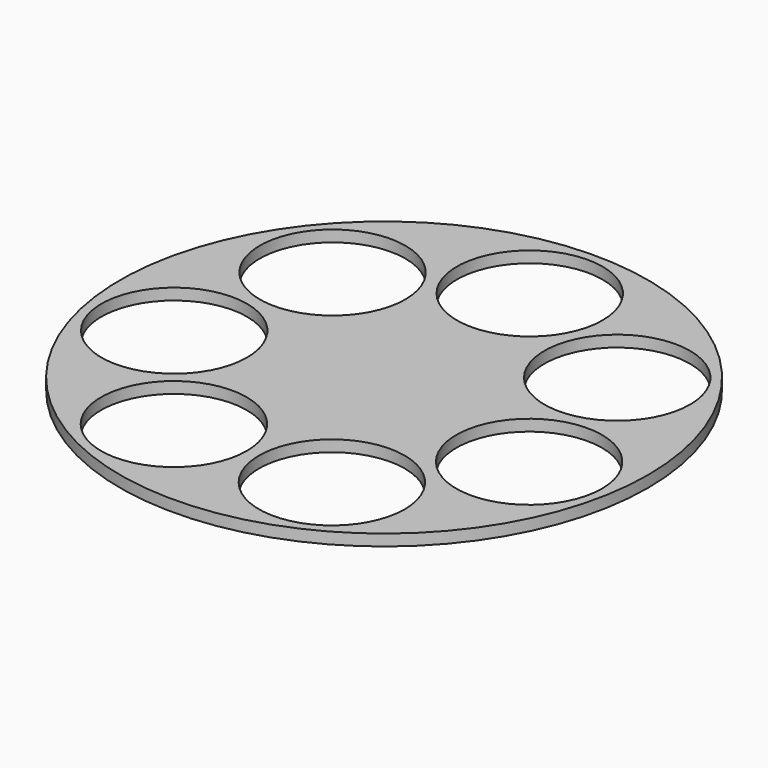
from build123d import *

# Parameters (mm, degrees)
F0_R     = 116
F0_R_2   = 32
F2_DEPTH = 5


# Not quite as in the source:
# - the program builds the solid bodies; features that only make, move or delete a surface that nothing else refers to are left out


with BuildPart() as f2:
    # F0 (on Top) → F2 (new body)
    with BuildSketch(Plane.XY):
        Circle(F0_R)
        with Locations((-34.7106991294, -72.0775094322)):
            Circle(F0_R_2, mode=Mode.SUBTRACT)
        with Locations((-77.9942329745, -17.8016747165)):
            Circle(F0_R_2, mode=Mode.SUBTRACT)
        with Locations((34.7106991294, -72.0775094322)):
            Circle(F0_R_2, mode=Mode.SUBTRACT)
        with Locations((77.9942329745, -17.8016747165)):
            Circle(F0_R_2, mode=Mode.SUBTRACT)
        with Locations((-62.5465185974, 49.8791841487)):
            Circle(F0_R_2, mode=Mode.SUBTRACT)
        with Locations((62.5465185974, 49.8791841487)):
            Circle(F0_R_2, mode=Mode.SUBTRACT)
        with Locations((0, 80)):
            Circle(F0_R_2, mode=Mode.SUBTRACT)
    extrude(amount=F2_DEPTH)


solid = f2.part
